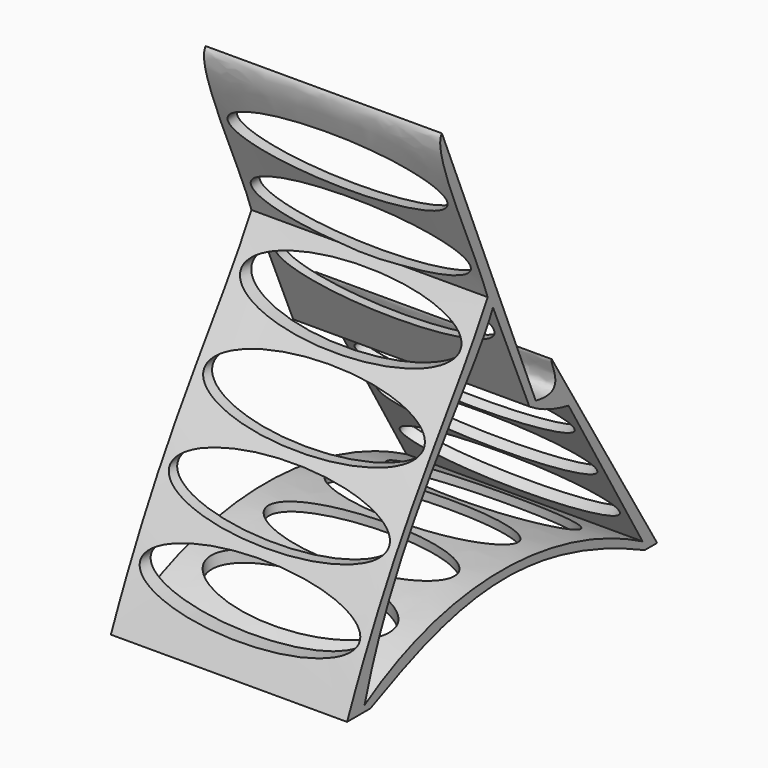
from build123d import *

# Parameters (mm, degrees)
F1_DEPTH  = 70
F3_REACH  = 140.8427948945
F5_REACH  = 198.6043545962
F8_REACH  = 187.2157962538
F9_REACH  = 187.2157962538
F12_REACH = 200.5256779964


# Not quite as in the source:
# - a feature names something its author has since deleted; it is built from what else it names


with BuildPart() as f1:
    # F0 (on Right) → F1 (new body)
    with BuildSketch(Plane.YZ):
        with BuildLine():
            Line((-65.0536715984, 0), (-56.4117916499, 0))
            add(Edge.make_bspline(
                [(-56.4117916499, 0), (-27.936052531, 13.126176782), (-1.7122571589, 22.8152908385), (45.2086254954, 0)],
                knots=[0, 0, 0, 0, 101.6204171453, 101.6204171453, 101.6204171453, 101.6204171453], degree=3))
            Line((45.2086254954, 0), (49.8031899333, 0))
            add(Edge.make_bspline(
                [(49.8031899333, 0), (36.7837014298, 21.2773953875), (23.7642129262, 42.554790775), (10.7447244227, 63.8321861625)],
                knots=[0, 0, 0, 0, 74.8338941812, 74.8338941812, 74.8338941812, 74.8338941812], degree=3))
            add(Edge.make_bspline(
                [(4.8285723044, 55.386091928), (17.0853175535, 52.8970839186), (9.9300900474, 62.5007674098), (10.7447244227, 63.8321861625)],
                knots=[0, 0, 0, 0, 10.3120009554, 10.3120009554, 10.3120009554, 10.3120009554], degree=3))
            Line((4.8285723044, 55.386091928), (-29.9188829958, 139.2738819122))
            add(Edge.make_bspline(
                [(-29.9188829958, 139.2738819122), (-33.9768491685, 135.0895613432), (-17.3589422678, 103.2935107748), (-12.9886427894, 89.6528437734)],
                knots=[0, 0, 0, 0, 52.4297669213, 52.4297669213, 52.4297669213, 52.4297669213], degree=3))
            add(Edge.make_bspline(
                [(-12.9886427894, 89.6528437734), (-26.6396608204, 64.4889175892), (-45.0603142381, 46.8906201422), (-65.0536715984, 0)],
                knots=[0, 0, 0, 0, 103.6744887691, 103.6744887691, 103.6744887691, 103.6744887691], degree=3))
        make_face()
        with BuildLine():
            add(Edge.make_bspline(
                [(-58.5831403732, 1.7520016991), (-26.5599957202, 21.9477838837), (12.6107810065, 19.9717469513), (44.4163493812, 2.5945331436)],
                knots=[0, 0, 0, 0, 103.0029356325, 103.0029356325, 103.0029356325, 103.0029356325], degree=3))
            add(Edge.make_bspline(
                [(-58.5831403732, 1.7520016991), (-46.7050112784, 43.4367507696), (-17.9227450863, 70.4098418355), (-11.0150016844, 86.1989706755)],
                knots=[0, 0, 0, 0, 96.9227444288, 96.9227444288, 96.9227444288, 96.9227444288], degree=3))
            Line((-11.0150016844, 86.1989706755), (2.4867416879, 54.8259804102))
            add(Edge.make_bspline(
                [(2.4867416879, 54.8259804102), (6.9520277902, 51.7374575138), (13.1526212381, 49.8405049891), (16.9847030193, 49.1881705821)],
                knots=[0, 0, 0, 0, 15.5555707843, 15.5555707843, 15.5555707843, 15.5555707843], degree=3))
            Line((16.9847030193, 49.1881705821), (44.4163493812, 2.5945331436))
        make_face(mode=Mode.SUBTRACT)
    extrude(amount=F1_DEPTH)

    f3_end = f1.faces().sort_by_distance((35, 30.273957178, 31.9160930812))[0]
    # F2 (on face) → F3 (cut, up to a face of the model that its end follows)
    with BuildSketch(Plane(origin=(0, 34.1179734072, 20.086694934), x_dir=(1, 0, 0), z_dir=(0, -0.8617432082, -0.5073446986))):
        with BuildLine():
            add(Edge.make_bspline(
                [(67.5, 23.4277807176), (67.5, 36.9762650043), (18.75, 30.202022861), (-30, 23.4277807176), (18.75, 16.6535385743), (67.5, 9.8792964309), (67.5, 23.4277807176)],
                knots=[0, 0, 0, 2.0943951024, 2.0943951024, 4.1887902048, 4.1887902048, 6.2831853072, 6.2831853072, 6.2831853072], degree=2, weights=[1, 0.5, 1, 0.5, 1, 0.5, 1]))
        make_face()
        with BuildLine():
            add(Edge.make_bspline(
                [(67.5, 6.9277807176), (67.5, 20.4762650043), (18.75, 13.702022861), (-30, 6.9277807176), (18.75, 0.1535385743), (67.5, -6.6207035691), (67.5, 6.9277807176)],
                knots=[0, 0, 0, 2.0943951024, 2.0943951024, 4.1887902048, 4.1887902048, 6.2831853072, 6.2831853072, 6.2831853072], degree=2, weights=[1, 0.5, 1, 0.5, 1, 0.5, 1]))
        make_face()
        with BuildLine():
            add(Edge.make_bspline(
                [(67.5, -9.5722192824), (67.5, 3.9762650043), (18.75, -2.797977139), (-30, -9.5722192824), (18.75, -16.3464614257), (67.5, -23.1207035691), (67.5, -9.5722192824)],
                knots=[0, 0, 0, 2.0943951024, 2.0943951024, 4.1887902048, 4.1887902048, 6.2831853072, 6.2831853072, 6.2831853072], degree=2, weights=[1, 0.5, 1, 0.5, 1, 0.5, 1]))
        make_face()
    f3_long = extrude(amount=-F3_REACH, mode=Mode.PRIVATE)
    add(split(f3_long, bisect_by=f3_end, keep=Keep.BOTTOM, mode=Mode.PRIVATE), mode=Mode.SUBTRACT)

    f5_end = f1.faces().sort_by_distance((35, -7.0018043916, 16.2631409185))[0]
    # F4 (on Top) → F5 (cut, up to a face of the model that its end follows)
    with BuildSketch(Plane.XY):
        with BuildLine():
            add(Edge.make_bspline(
                [(62.8528258204, -38.5428890586), (62.8528258204, -20.8609774983), (21.0735870898, -29.7019332784), (-20.7056516409, -38.5428890586), (21.0735870898, -47.3838448388), (62.8528258204, -56.2248006189), (62.8528258204, -38.5428890586)],
                knots=[0, 0, 0, 2.0943951024, 2.0943951024, 4.1887902048, 4.1887902048, 6.2831853072, 6.2831853072, 6.2831853072], degree=2, weights=[1, 0.5, 1, 0.5, 1, 0.5, 1]))
        make_face()
        with BuildLine():
            add(Edge.make_bspline(
                [(62.8528258204, -15.9428890586), (62.8528258204, 1.7390225017), (21.0735870898, -7.1019332784), (-20.7056516409, -15.9428890586), (21.0735870898, -24.7838448388), (62.8528258204, -33.6248006189), (62.8528258204, -15.9428890586)],
                knots=[0, 0, 0, 2.0943951024, 2.0943951024, 4.1887902048, 4.1887902048, 6.2831853072, 6.2831853072, 6.2831853072], degree=2, weights=[1, 0.5, 1, 0.5, 1, 0.5, 1]))
        make_face()
        with BuildLine():
            add(Edge.make_bspline(
                [(62.8528258204, 6.6571109414), (62.8528258204, 24.3390225017), (21.0735870898, 15.4980667216), (-20.7056516409, 6.6571109414), (21.0735870898, -2.1838448388), (62.8528258204, -11.0248006189), (62.8528258204, 6.6571109414)],
                knots=[0, 0, 0, 2.0943951024, 2.0943951024, 4.1887902048, 4.1887902048, 6.2831853072, 6.2831853072, 6.2831853072], degree=2, weights=[1, 0.5, 1, 0.5, 1, 0.5, 1]))
        make_face()
        with BuildLine():
            add(Edge.make_bspline(
                [(62.8528258204, 29.2571109414), (62.8528258204, 46.9390225017), (21.0735870898, 38.0980667216), (-20.7056516409, 29.2571109414), (21.0735870898, 20.4161551612), (62.8528258204, 11.5751993811), (62.8528258204, 29.2571109414)],
                knots=[0, 0, 0, 2.0943951024, 2.0943951024, 4.1887902048, 4.1887902048, 6.2831853072, 6.2831853072, 6.2831853072], degree=2, weights=[1, 0.5, 1, 0.5, 1, 0.5, 1]))
        make_face()
    f5_long = extrude(amount=F5_REACH, mode=Mode.PRIVATE)
    add(split(f5_long, bisect_by=f5_end, keep=Keep.BOTTOM, mode=Mode.PRIVATE), mode=Mode.SUBTRACT)

    f8_end = f1.faces().sort_by_distance((35, -32.9351763939, 53.6863437737))[0]
    # F7 (on offset) → F8 (cut, up to a face of the model that its end follows)
    with BuildSketch(Plane.XZ.offset(70)):
        with BuildLine():
            add(Edge.make_bspline(
                [(67.5, 57.6202747583), (67.5, 73.0958511632), (18.75, 65.3580629608), (-30, 57.6202747583), (18.75, 49.8824865559), (67.5, 42.1446983534), (67.5, 57.6202747583)],
                knots=[0, 0, 0, 2.0943951024, 2.0943951024, 4.1887902048, 4.1887902048, 6.2831853072, 6.2831853072, 6.2831853072], degree=2, weights=[1, 0.5, 1, 0.5, 1, 0.5, 1]))
        make_face()
        with BuildLine():
            add(Edge.make_bspline(
                [(67.5, 37.3202747583), (67.5, 52.7958511632), (18.75, 45.0580629608), (-30, 37.3202747583), (18.75, 29.5824865559), (67.5, 21.8446983534), (67.5, 37.3202747583)],
                knots=[0, 0, 0, 2.0943951024, 2.0943951024, 4.1887902048, 4.1887902048, 6.2831853072, 6.2831853072, 6.2831853072], degree=2, weights=[1, 0.5, 1, 0.5, 1, 0.5, 1]))
        make_face()
        with BuildLine():
            add(Edge.make_bspline(
                [(67.5, 17.0202747583), (67.5, 32.4958511632), (18.75, 24.7580629608), (-30, 17.0202747583), (18.75, 9.2824865559), (67.5, 1.5446983534), (67.5, 17.0202747583)],
                knots=[0, 0, 0, 2.0943951024, 2.0943951024, 4.1887902048, 4.1887902048, 6.2831853072, 6.2831853072, 6.2831853072], degree=2, weights=[1, 0.5, 1, 0.5, 1, 0.5, 1]))
        make_face()
    f8_long = extrude(amount=-F8_REACH, mode=Mode.PRIVATE)
    add(split(f8_long, bisect_by=f8_end, keep=Keep.BOTTOM, mode=Mode.PRIVATE), mode=Mode.SUBTRACT)

    f9_end = f1.faces().sort_by_distance((35, -12.5451553457, 97.3299869201))[0]
    # F7 (on offset) → F9 (cut, up to a face of the model that its end follows)
    with BuildSketch(Plane.XZ.offset(70)):
        with BuildLine():
            add(Edge.make_bspline(
                [(67.5, 118.5202747583), (67.5, 133.9958511632), (18.75, 126.2580629608), (-30, 118.5202747583), (18.75, 110.7824865559), (67.5, 103.0446983534), (67.5, 118.5202747583)],
                knots=[0, 0, 0, 2.0943951024, 2.0943951024, 4.1887902048, 4.1887902048, 6.2831853072, 6.2831853072, 6.2831853072], degree=2, weights=[1, 0.5, 1, 0.5, 1, 0.5, 1]))
        make_face()
        with BuildLine():
            add(Edge.make_bspline(
                [(67.5, 98.2202747583), (67.5, 113.6958511632), (18.75, 105.9580629608), (-30, 98.2202747583), (18.75, 90.4824865559), (67.5, 82.7446983534), (67.5, 98.2202747583)],
                knots=[0, 0, 0, 2.0943951024, 2.0943951024, 4.1887902048, 4.1887902048, 6.2831853072, 6.2831853072, 6.2831853072], degree=2, weights=[1, 0.5, 1, 0.5, 1, 0.5, 1]))
        make_face()
        with BuildLine():
            add(Edge.make_bspline(
                [(67.5, 77.9202747583), (67.5, 93.3958511632), (18.75, 85.6580629608), (-30, 77.9202747583), (18.75, 70.1824865559), (67.5, 62.4446983534), (67.5, 77.9202747583)],
                knots=[0, 0, 0, 2.0943951024, 2.0943951024, 4.1887902048, 4.1887902048, 6.2831853072, 6.2831853072, 6.2831853072], degree=2, weights=[1, 0.5, 1, 0.5, 1, 0.5, 1]))
        make_face()
    f9_long = extrude(amount=-F9_REACH, mode=Mode.PRIVATE)
    add(split(f9_long, bisect_by=f9_end, keep=Keep.BOTTOM, mode=Mode.PRIVATE), mode=Mode.SUBTRACT)

    f12_end = f1.faces().sort_by_distance((35, 9.973173974, 51.0935048126))[0]
    # F11 (on face) → F12 (cut, up to a face of the model that its end follows)
    with BuildSketch(Plane(origin=(0, -53.6222660217, 129.4556206097), x_dir=(1, 0, 0), z_dir=(0, -0.3826833851, 0.9238795521))):
        with BuildLine():
            add(Edge.make_bspline(
                [(14.718651472, 29.656356364), (14.718651472, 22.7281531337), (45.140674264, 26.1922547488), (75.562697056, 29.656356364), (45.140674264, 33.1204579791), (14.718651472, 36.5845595942), (14.718651472, 29.656356364)],
                knots=[0, 0, 0, 2.0943951024, 2.0943951024, 4.1887902048, 4.1887902048, 6.2831853072, 6.2831853072, 6.2831853072], degree=2, weights=[1, 0.5, 1, 0.5, 1, 0.5, 1]))
        make_face()
    f12_long = extrude(amount=-F12_REACH, mode=Mode.PRIVATE)
    add(split(f12_long, bisect_by=f12_end, keep=Keep.BOTTOM, mode=Mode.PRIVATE), mode=Mode.SUBTRACT)


solid = f1.part
